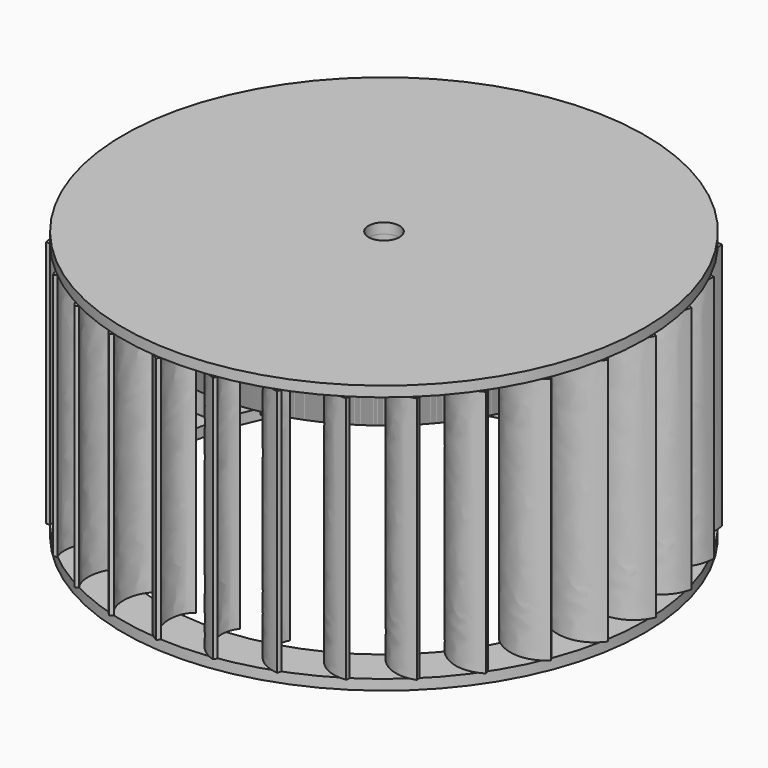
from build123d import *

# Parameters (mm, degrees)
F0_R      = 40.5
F1_DEPTH  = 10
F3_DEPTH  = 48
F5_COUNT  = 30
F6_R      = 50.5
F7_DEPTH  = 2
F8_R      = 50.5
F8_R_2    = 42.5
F9_DEPTH  = 2
F10_R     = 3
F11_DEPTH = 52.001
F12_R     = 3
F13_DEPTH = 25


with BuildPart() as f1:
    # F0 (on Top) → F1 (new body)
    with BuildSketch(Plane.XY):
        Circle(F0_R)
    extrude(amount=F1_DEPTH)

    # F2 (on face) → F3 (join)
    with BuildSketch(Plane.XY.offset(10)):
        with BuildLine():
            add(Edge.make_bspline(
                [(20.1993929166, 35.1031982275), (23.6904856829, 35.8287255413), (25.615372677, 41.7569810201), (23.1102083027, 44.9017624621)],
                knots=[0, 0, 0, 0, 10.221776131, 10.221776131, 10.221776131, 10.221776131], degree=3))
            ThreePointArc((20.1993929166, 35.1031982275), (20.7205022018, 34.7981434635), (21.2370054998, 34.4853533751))
            add(Edge.make_bspline(
                [(23.8099146315, 45.2130903834), (27.6339743286, 40.0055646896), (22.8687301278, 34.5244519413), (21.2370054998, 34.4853533751)],
                knots=[0, 0, 0, 0, 11.0319627773, 11.0319627773, 11.0319627773, 11.0319627773], degree=3))
            Line((23.8099146315, 45.2130903834), (23.1102083027, 44.9017624621))
        make_face()
    extrude(amount=-F3_DEPTH)


with BuildPart() as f5_1:
    # F5: instance of F1
    add(f1.part.rotate(Axis((0, 0, 0), (0, 0, -1)), 1 * 360 / F5_COUNT))


with BuildPart() as f5_2:
    # F5: instance of F1
    add(f1.part.rotate(Axis((0, 0, 0), (0, 0, -1)), 2 * 360 / F5_COUNT))


with BuildPart() as f5_3:
    # F5: instance of F1
    add(f1.part.rotate(Axis((0, 0, 0), (0, 0, -1)), 3 * 360 / F5_COUNT))


with BuildPart() as f5_4:
    # F5: instance of F1
    add(f1.part.rotate(Axis((0, 0, 0), (0, 0, -1)), 4 * 360 / F5_COUNT))


with BuildPart() as f5_5:
    # F5: instance of F1
    add(f1.part.rotate(Axis((0, 0, 0), (0, 0, -1)), 5 * 360 / F5_COUNT))


with BuildPart() as f5_6:
    # F5: instance of F1
    add(f1.part.rotate(Axis((0, 0, 0), (0, 0, -1)), 6 * 360 / F5_COUNT))


with BuildPart() as f5_7:
    # F5: instance of F1
    add(f1.part.rotate(Axis((0, 0, 0), (0, 0, -1)), 7 * 360 / F5_COUNT))


with BuildPart() as f5_8:
    # F5: instance of F1
    add(f1.part.rotate(Axis((0, 0, 0), (0, 0, -1)), 8 * 360 / F5_COUNT))


with BuildPart() as f5_9:
    # F5: instance of F1
    add(f1.part.rotate(Axis((0, 0, 0), (0, 0, -1)), 9 * 360 / F5_COUNT))


with BuildPart() as f5_10:
    # F5: instance of F1
    add(f1.part.rotate(Axis((0, 0, 0), (0, 0, -1)), 10 * 360 / F5_COUNT))


with BuildPart() as f5_11:
    # F5: instance of F1
    add(f1.part.rotate(Axis((0, 0, 0), (0, 0, -1)), 11 * 360 / F5_COUNT))


with BuildPart() as f5_12:
    # F5: instance of F1
    add(f1.part.rotate(Axis((0, 0, 0), (0, 0, -1)), 12 * 360 / F5_COUNT))


with BuildPart() as f5_13:
    # F5: instance of F1
    add(f1.part.rotate(Axis((0, 0, 0), (0, 0, -1)), 13 * 360 / F5_COUNT))


with BuildPart() as f5_14:
    # F5: instance of F1
    add(f1.part.rotate(Axis((0, 0, 0), (0, 0, -1)), 14 * 360 / F5_COUNT))


with BuildPart() as f5_15:
    # F5: instance of F1
    add(f1.part.rotate(Axis((0, 0, 0), (0, 0, -1)), 15 * 360 / F5_COUNT))


with BuildPart() as f5_16:
    # F5: instance of F1
    add(f1.part.rotate(Axis((0, 0, 0), (0, 0, -1)), 16 * 360 / F5_COUNT))


with BuildPart() as f5_17:
    # F5: instance of F1
    add(f1.part.rotate(Axis((0, 0, 0), (0, 0, -1)), 17 * 360 / F5_COUNT))


with BuildPart() as f5_18:
    # F5: instance of F1
    add(f1.part.rotate(Axis((0, 0, 0), (0, 0, -1)), 18 * 360 / F5_COUNT))


with BuildPart() as f5_19:
    # F5: instance of F1
    add(f1.part.rotate(Axis((0, 0, 0), (0, 0, -1)), 19 * 360 / F5_COUNT))


with BuildPart() as f5_20:
    # F5: instance of F1
    add(f1.part.rotate(Axis((0, 0, 0), (0, 0, -1)), 20 * 360 / F5_COUNT))


with BuildPart() as f5_21:
    # F5: instance of F1
    add(f1.part.rotate(Axis((0, 0, 0), (0, 0, -1)), 21 * 360 / F5_COUNT))


with BuildPart() as f5_22:
    # F5: instance of F1
    add(f1.part.rotate(Axis((0, 0, 0), (0, 0, -1)), 22 * 360 / F5_COUNT))


with BuildPart() as f5_23:
    # F5: instance of F1
    add(f1.part.rotate(Axis((0, 0, 0), (0, 0, -1)), 23 * 360 / F5_COUNT))


with BuildPart() as f5_24:
    # F5: instance of F1
    add(f1.part.rotate(Axis((0, 0, 0), (0, 0, -1)), 24 * 360 / F5_COUNT))


with BuildPart() as f5_25:
    # F5: instance of F1
    add(f1.part.rotate(Axis((0, 0, 0), (0, 0, -1)), 25 * 360 / F5_COUNT))


with BuildPart() as f5_26:
    # F5: instance of F1
    add(f1.part.rotate(Axis((0, 0, 0), (0, 0, -1)), 26 * 360 / F5_COUNT))


with BuildPart() as f5_27:
    # F5: instance of F1
    add(f1.part.rotate(Axis((0, 0, 0), (0, 0, -1)), 27 * 360 / F5_COUNT))


with BuildPart() as f5_28:
    # F5: instance of F1
    add(f1.part.rotate(Axis((0, 0, 0), (0, 0, -1)), 28 * 360 / F5_COUNT))


with BuildPart() as f5_29:
    # F5: instance of F1
    add(f1.part.rotate(Axis((0, 0, 0), (0, 0, -1)), 29 * 360 / F5_COUNT))


with BuildPart() as f7:
    # F6 (on face) → F7 (new body)
    with BuildSketch(Plane.XY.offset(10)):
        Circle(F6_R)
    extrude(amount=F7_DEPTH)


with BuildPart() as f9:
    # F8 (on face) → F9 (new body)
    with BuildSketch(Plane(origin=(0, 0, -38), x_dir=(1, 0, 0), z_dir=(0, 0, -1))):
        Circle(F8_R)
        Circle(F8_R_2, mode=Mode.SUBTRACT)
    extrude(amount=F9_DEPTH)


with BuildPart() as f11_tool:
    # F10 (on face) → F11 (new body, through all)
    with BuildSketch(Plane.XY.offset(12)):
        Circle(F10_R)
    extrude(amount=-F11_DEPTH)


with BuildPart() as f1_1:
    add(f1.part)

    # F11: cut by f11_tool
    add(f11_tool.part, mode=Mode.SUBTRACT)

    # F12 (on face) → F13 (cut)
    with BuildSketch(Plane(origin=(0, 0, 0), x_dir=(1, 0, 0), z_dir=(0, 0, -1))):
        Circle(F12_R)
    extrude(amount=-F13_DEPTH, mode=Mode.SUBTRACT)


with BuildPart() as f5_1_1:
    add(f5_1.part)

    # F11: cut by f11_tool
    add(f11_tool.part, mode=Mode.SUBTRACT)


with BuildPart() as f5_2_1:
    add(f5_2.part)

    # F11: cut by f11_tool
    add(f11_tool.part, mode=Mode.SUBTRACT)


with BuildPart() as f5_3_1:
    add(f5_3.part)

    # F11: cut by f11_tool
    add(f11_tool.part, mode=Mode.SUBTRACT)


with BuildPart() as f5_4_1:
    add(f5_4.part)

    # F11: cut by f11_tool
    add(f11_tool.part, mode=Mode.SUBTRACT)


with BuildPart() as f5_5_1:
    add(f5_5.part)

    # F11: cut by f11_tool
    add(f11_tool.part, mode=Mode.SUBTRACT)


with BuildPart() as f5_6_1:
    add(f5_6.part)

    # F11: cut by f11_tool
    add(f11_tool.part, mode=Mode.SUBTRACT)


with BuildPart() as f5_7_1:
    add(f5_7.part)

    # F11: cut by f11_tool
    add(f11_tool.part, mode=Mode.SUBTRACT)


with BuildPart() as f5_8_1:
    add(f5_8.part)

    # F11: cut by f11_tool
    add(f11_tool.part, mode=Mode.SUBTRACT)


with BuildPart() as f5_9_1:
    add(f5_9.part)

    # F11: cut by f11_tool
    add(f11_tool.part, mode=Mode.SUBTRACT)


with BuildPart() as f5_10_1:
    add(f5_10.part)

    # F11: cut by f11_tool
    add(f11_tool.part, mode=Mode.SUBTRACT)


with BuildPart() as f5_11_1:
    add(f5_11.part)

    # F11: cut by f11_tool
    add(f11_tool.part, mode=Mode.SUBTRACT)


with BuildPart() as f5_12_1:
    add(f5_12.part)

    # F11: cut by f11_tool
    add(f11_tool.part, mode=Mode.SUBTRACT)


with BuildPart() as f5_13_1:
    add(f5_13.part)

    # F11: cut by f11_tool
    add(f11_tool.part, mode=Mode.SUBTRACT)


with BuildPart() as f5_14_1:
    add(f5_14.part)

    # F11: cut by f11_tool
    add(f11_tool.part, mode=Mode.SUBTRACT)


with BuildPart() as f5_15_1:
    add(f5_15.part)

    # F11: cut by f11_tool
    add(f11_tool.part, mode=Mode.SUBTRACT)


with BuildPart() as f5_16_1:
    add(f5_16.part)

    # F11: cut by f11_tool
    add(f11_tool.part, mode=Mode.SUBTRACT)


with BuildPart() as f5_17_1:
    add(f5_17.part)

    # F11: cut by f11_tool
    add(f11_tool.part, mode=Mode.SUBTRACT)


with BuildPart() as f5_18_1:
    add(f5_18.part)

    # F11: cut by f11_tool
    add(f11_tool.part, mode=Mode.SUBTRACT)


with BuildPart() as f5_19_1:
    add(f5_19.part)

    # F11: cut by f11_tool
    add(f11_tool.part, mode=Mode.SUBTRACT)


with BuildPart() as f5_20_1:
    add(f5_20.part)

    # F11: cut by f11_tool
    add(f11_tool.part, mode=Mode.SUBTRACT)


with BuildPart() as f5_21_1:
    add(f5_21.part)

    # F11: cut by f11_tool
    add(f11_tool.part, mode=Mode.SUBTRACT)


with BuildPart() as f5_22_1:
    add(f5_22.part)

    # F11: cut by f11_tool
    add(f11_tool.part, mode=Mode.SUBTRACT)


with BuildPart() as f5_23_1:
    add(f5_23.part)

    # F11: cut by f11_tool
    add(f11_tool.part, mode=Mode.SUBTRACT)


with BuildPart() as f5_24_1:
    add(f5_24.part)

    # F11: cut by f11_tool
    add(f11_tool.part, mode=Mode.SUBTRACT)


with BuildPart() as f5_25_1:
    add(f5_25.part)

    # F11: cut by f11_tool
    add(f11_tool.part, mode=Mode.SUBTRACT)


with BuildPart() as f5_26_1:
    add(f5_26.part)

    # F11: cut by f11_tool
    add(f11_tool.part, mode=Mode.SUBTRACT)


with BuildPart() as f5_27_1:
    add(f5_27.part)

    # F11: cut by f11_tool
    add(f11_tool.part, mode=Mode.SUBTRACT)


with BuildPart() as f5_28_1:
    add(f5_28.part)

    # F11: cut by f11_tool
    add(f11_tool.part, mode=Mode.SUBTRACT)


with BuildPart() as f5_29_1:
    add(f5_29.part)

    # F11: cut by f11_tool
    add(f11_tool.part, mode=Mode.SUBTRACT)


with BuildPart() as f7_1:
    add(f7.part)

    # F11: cut by f11_tool
    add(f11_tool.part, mode=Mode.SUBTRACT)


solid = Compound([f9.part, f1_1.part, f5_1_1.part, f5_2_1.part, f5_3_1.part, f5_4_1.part, f5_5_1.part, f5_6_1.part, f5_7_1.part, f5_8_1.part, f5_9_1.part, f5_10_1.part, f5_11_1.part, f5_12_1.part, f5_13_1.part, f5_14_1.part, f5_15_1.part, f5_16_1.part, f5_17_1.part, f5_18_1.part, f5_19_1.part, f5_20_1.part, f5_21_1.part, f5_22_1.part, f5_23_1.part, f5_24_1.part, f5_25_1.part, f5_26_1.part, f5_27_1.part, f5_28_1.part, f5_29_1.part, f7_1.part])
